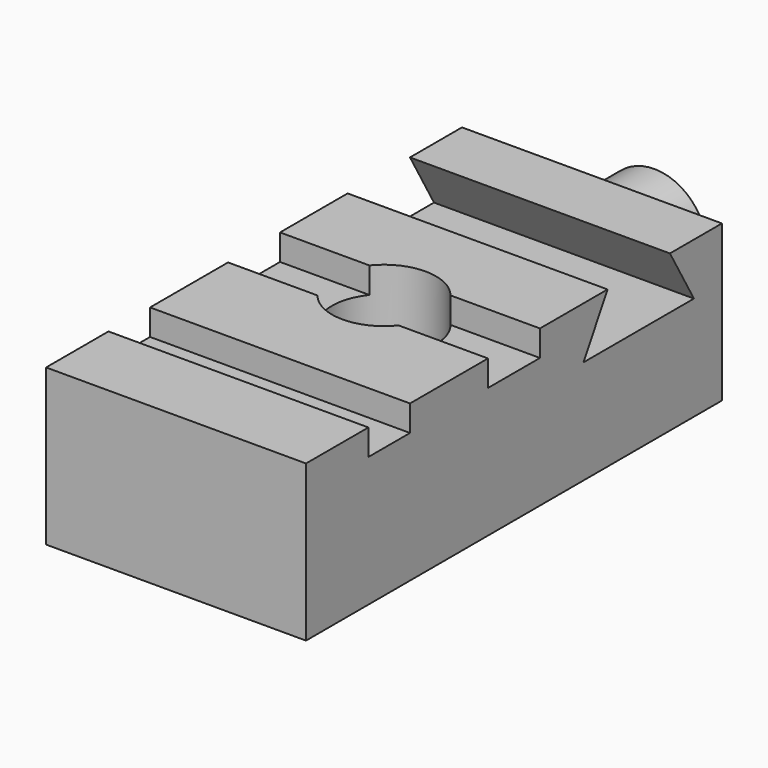
from build123d import *

# Parameters (mm, degrees)
F0_W     = 50
F0_H     = 100
F0_R     = 10
F1_DEPTH = 30
F2_W     = 50
F2_H     = 10
F3_DEPTH = 5
F5_DEPTH = 50
F6_R     = 10
F7_DEPTH = 15


with BuildPart() as f1:
    # F0 (on Top) → F1 (new body)
    with BuildSketch(Plane.XY):
        Rectangle(F0_W, F0_H)
        Circle(F0_R, mode=Mode.SUBTRACT)
    extrude(amount=F1_DEPTH)

    # F2 (on face) → F3 (cut)
    with BuildSketch(Plane.XY.offset(30)):
        with BuildLine():
            Line((7.806247498, -6.25), (25, -6.25))
            Line((25, -6.25), (25, 6.25))
            Line((25, 6.25), (7.806247498, 6.25))
            ThreePointArc((7.806247498, 6.25), (9.4356365705, 3.3119122135), (10, 0))
            ThreePointArc((10, 0), (9.4356365705, -3.3119122135), (7.806247498, -6.25))
        make_face()
        with Locations((0, -30)):
            Rectangle(F2_W, F2_H)
        with BuildLine():
            Line((-25, 6.25), (-25, -6.25))
            Line((-25, -6.25), (-7.806247498, -6.25))
            ThreePointArc((-7.806247498, -6.25), (-10, 0), (-7.806247498, 6.25))
            Line((-7.806247498, 6.25), (-25, 6.25))
        make_face()
    extrude(amount=-F3_DEPTH, mode=Mode.SUBTRACT)

    # F4 (on face) → F5 (cut, through all)
    with BuildSketch(Plane(origin=(-25, 0, 0), x_dir=(0, -1, 0), z_dir=(-1, 0, 0))):
        Polygon((-22.5, 30), (-37.5, 30), (-43.2735026919, 20), (-16.7264973081, 20), align=None)
    extrude(amount=-F5_DEPTH, mode=Mode.SUBTRACT)

    # F6 (on face) → F7 (join)
    with BuildSketch(Plane(origin=(0, 50, 0), x_dir=(-1, 0, 0), z_dir=(0, 1, 0))):
        with Locations((0, 15)):
            Circle(F6_R)
    extrude(amount=F7_DEPTH)


solid = f1.part
